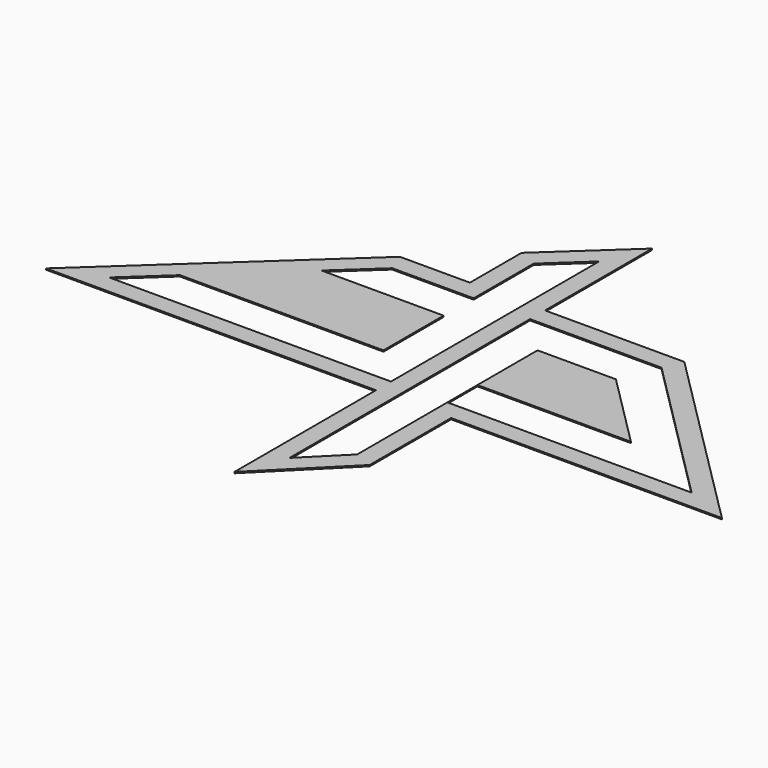
from build123d import *

# Parameters (mm, degrees)
F0_W     = 0.001
F0_H     = 60
F1_DEPTH = 2


with BuildPart() as f1:
    # F0 (on Top) → F1 (new body)
    with BuildSketch(Plane.XY):
        Polygon((-409.5329046249, 489.3550023332), (-409.5329046249, 703.2591700554), (-439.5329046249, 675.5668623631), (-439.5329046249, 634.7396177178), (-439.5329046249, 219.3550023332), (-439.5329046249, 189.3550023332), (-439.5329046249, -93.071404538), (-409.5329046249, -63.071404538), (-409.5329046249, -20.6449976668), (-409.5329046249, 189.3550023332), (-409.5329046249, 279.3550023332), (-409.5329046249, 399.3550023332), (-409.5329046249, 459.3550023332), align=None)
        Polygon((-187.1064977537, 489.3550023332), (-409.5329046249, 489.3550023332), (-409.5329046249, 459.3550023332), (-199.5329046249, 459.3550023332), (-157.1064977537, 459.3550023332), align=None)
        Polygon((-439.5329046249, 634.7396177178), (-439.5329046249, 675.5668623631), (-499.5329046249, 620.1822469785), (-499.5329046249, 579.3550023332), align=None)
        Polygon((-499.5329046249, 579.3550023332), (-499.5329046249, 620.1822469785), (-529.5329046249, 592.4899392862), (-529.5329046249, 551.6626946409), align=None)
        Polygon((-157.1064977537, 459.3550023332), (-199.5329046249, 459.3550023332), (-139.5329046249, 399.3550023332), (40.4670953751, 219.3550023332), (-44.3857183673, 219.3550023332), (-349.5319046249, 219.3550023332), (-349.5329046249, 219.3550023332), (-349.5329046249, 189.3550023332), (-319.5329046249, 189.3550023332), (112.8935022463, 189.3550023332), align=None)
        Polygon((-439.5329046249, 189.3550023332), (-439.5329046249, 219.3550023332), (-889.5329046249, 219.3550023332), (-922.0329046249, 189.3550023332), align=None)
        Polygon((-499.5329046249, 459.3550023332), (-499.5329046249, 579.3550023332), (-529.5329046249, 551.6626946409), (-529.5329046249, 489.3550023332), (-597.0329046249, 489.3550023332), (-629.5329046249, 459.3550023332), align=None)
        Polygon((-224.3857183673, 399.3550023332), (-349.5329046249, 399.3550023332), (-349.5329046249, 279.3550023332), (-349.5319046249, 279.3550023332), (-104.3857183673, 279.3550023332), align=None)
        Polygon((-922.0329046249, 189.3550023332), (-889.5329046249, 219.3550023332), (-933.7624196573, 219.3550023332), (-966.2624196573, 189.3550023332), align=None)
        Polygon((-933.7624196573, 219.3550023332), (-889.5329046249, 219.3550023332), (-824.5329046249, 279.3550023332), (-868.7624196573, 279.3550023332), align=None)
        Polygon((-597.0329046249, 489.3550023332), (-641.2624196573, 489.3550023332), (-673.7624196573, 459.3550023332), (-629.5329046249, 459.3550023332), align=None)
        with Locations((-349.5324046249, 249.3550023332)):
            Rectangle(F0_W, F0_H)
        Polygon((-319.5329046249, 26.928595462), (-319.5329046249, 189.3550023332), (-349.5329046249, 189.3550023332), (-349.5329046249, 39.3550023332), (-349.5329046249, -3.071404538), align=None)
        Polygon((-694.5329046249, 399.3550023332), (-824.5329046249, 279.3550023332), (-499.5329046249, 279.3550023332), (-499.5329046249, 399.3550023332), align=None)
        Polygon((-868.7624196573, 279.3550023332), (-824.5329046249, 279.3550023332), (-694.5329046249, 399.3550023332), (-738.7624196573, 399.3550023332), align=None)
        Polygon((-694.5329046249, 399.3550023332), (-629.5329046249, 459.3550023332), (-673.7624196573, 459.3550023332), (-738.7624196573, 399.3550023332), align=None)
        Polygon((-349.5329046249, 39.3550023332), (-409.5329046249, -20.6449976668), (-409.5329046249, -63.071404538), (-349.5329046249, -3.071404538), align=None)
    extrude(amount=F1_DEPTH)


solid = f1.part
